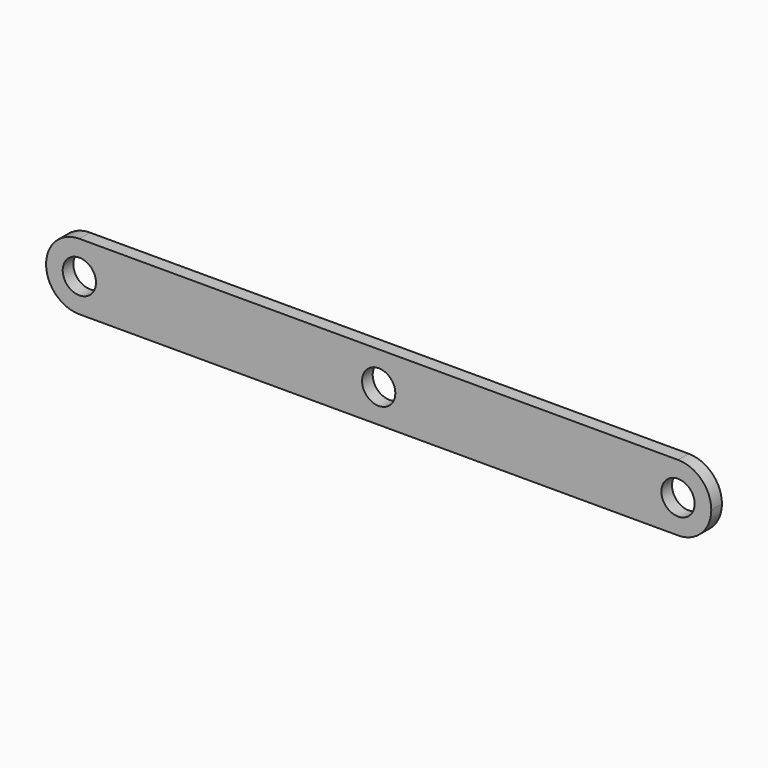
from build123d import *

# Parameters (mm, degrees)
F0_W     = 100
F0_H     = 10
F0_R     = 2.5
F1_DEPTH = 2
F2_R     = 4.99999


# Not quite as in the source:
# - a fillet or chamfer is up to 0.001 mm smaller than in the source, because OpenCascade refuses the exact size


with BuildPart() as f1:
    # F0 (on Front) → F1 (new body)
    with BuildSketch(Plane.XZ):
        Rectangle(F0_W, F0_H)
        with Locations((-45, 0)):
            Circle(F0_R, mode=Mode.SUBTRACT)
        Circle(F0_R, mode=Mode.SUBTRACT)
        with Locations((45, 0)):
            Circle(F0_R, mode=Mode.SUBTRACT)
    extrude(amount=F1_DEPTH)

    # F2 (radius 5 in the source; OpenCascade refuses exactly that, so slightly less here)
    f2_edges = [f1.edges().sort_by_distance(p)[0] for p in [
        (-50, -1, 5),
        (-50, -1, -5),
        (50, -1, -5),
        (50, -1, 5),
    ]]
    fillet(f2_edges, radius=F2_R)


with BuildPart() as f3_1:
    # F3: copy of F1
    add(f1.part.moved(Location((0, -2, 0))))


solid = f1.part
